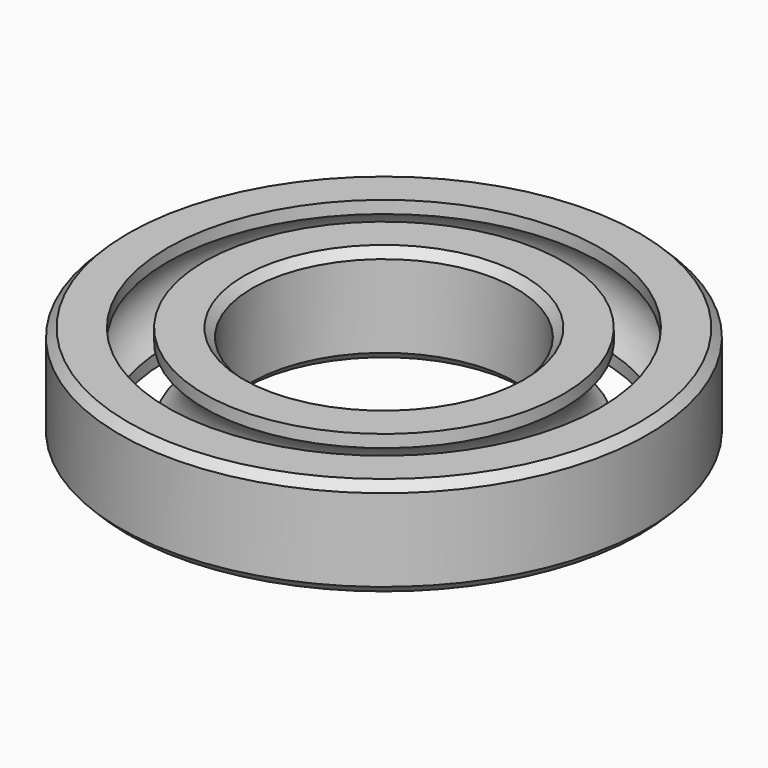
from build123d import *

# Parameters (mm, degrees)
F2_SIZE   = 1.5
F2_2_SIZE = 1.5


# Not quite as in the source:
# - a feature of the source that left no trace in its solid (it failed there, or was rolled back) is left out
# - the program builds the solid bodies; features that only make, move or delete a surface that nothing else refers to are left out


with BuildPart() as f1:
    # F0 (on Front) → F1 (revolve)
    with BuildSketch(Plane.XZ):
        with BuildLine():
            ThreePointArc((-39.3501091827, -6.7276512101), (-43.5156185601, 0), (-39.3501091827, 6.7276512101))
            Line((-39.3501091827, 6.7276512101), (-39.3501091827, 9))
            Line((-39.3501091827, 9), (-48, 9))
            Line((-48, 9), (-48, -9))
            Line((-48, -9), (-39.3501091827, -9))
            Line((-39.3501091827, -9), (-39.3501091827, -6.7276512101))
        make_face()
    revolve(axis=Axis((0, 0, -2.1557251625), (0, 0, -1)))

    # F2
    f2_edges = [f1.edges().sort_by_distance(p)[0] for p in [
        (48, 0, 9),
        (48, 0, -9),
    ]]
    chamfer(f2_edges, length=F2_SIZE)


with BuildPart() as f1b:
    # F0 (on Front) → F1, piece 2 (revolve)
    with BuildSketch(Plane.XZ):
        with BuildLine():
            Line((-24, 9), (-32.6498908173, 9))
            Line((-32.6498908173, 9), (-32.6498908173, 6.7276512101))
            ThreePointArc((-32.6498908173, 6.7276512101), (-28.4843814399, 0), (-32.6498908173, -6.7276512101))
            Line((-32.6498908173, -6.7276512101), (-32.6498908173, -9))
            Line((-32.6498908173, -9), (-24, -9))
            Line((-24, -9), (-24, 9))
        make_face()
    revolve(axis=Axis((0, 0, -2.1557251625), (0, 0, -1)))

    # F2#2
    f2_2_edges = [f1b.edges().sort_by_distance(p)[0] for p in [
        (24, 0, 9),
        (24, 0, -9),
    ]]
    chamfer(f2_2_edges, length=F2_2_SIZE)


solid = Compound([f1.part, f1b.part])
